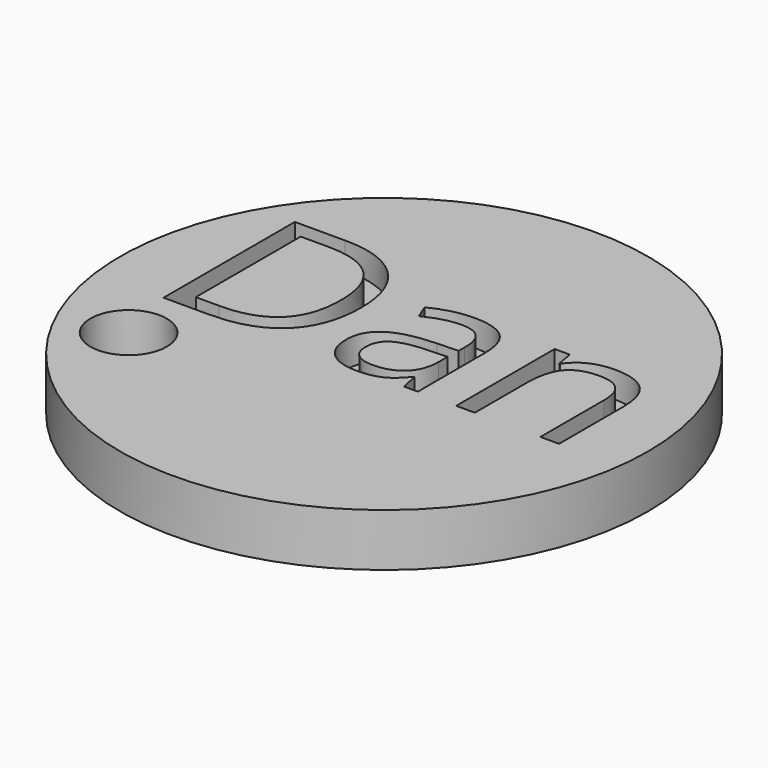
from build123d import *

# Parameters (mm, degrees)
F0_R         = 30
F1_DEPTH     = 3
F2_R         = 4.3372023121
F3_DEPTH     = 6
F4_TEXT_SIZE = 26.1314653067
F5_DEPTH     = 3


# Not quite as in the source:
# - Text() gives the source's letters only with a copy of the font that has no kerning and outlines rounded to 1/6400 em; it was checked with that copy


with BuildPart() as f1:
    # F0 (on Top) → F1 (new body, symmetric)
    with BuildSketch(Plane.XY):
        Circle(F0_R)
    extrude(amount=F1_DEPTH, both=True)

    # F2 (on face) → F3 (cut)
    with BuildSketch(Plane.XY.offset(3)):
        with Locations((-20.2693976462, -10.9590515494)):
            Circle(F2_R)
    extrude(amount=-F3_DEPTH, mode=Mode.SUBTRACT)

    # F4 (on face) → F5 (cut)
    with BuildSketch(Plane.XY.offset(3)):
        with Locations((-24.6064493236, -3.7823272869)):
            Text('Dan', F4_TEXT_SIZE, font='Open Sans', text_align=(TextAlign.LEFT, TextAlign.BOTTOM))
    extrude(amount=-F5_DEPTH, mode=Mode.SUBTRACT)


solid = f1.part
